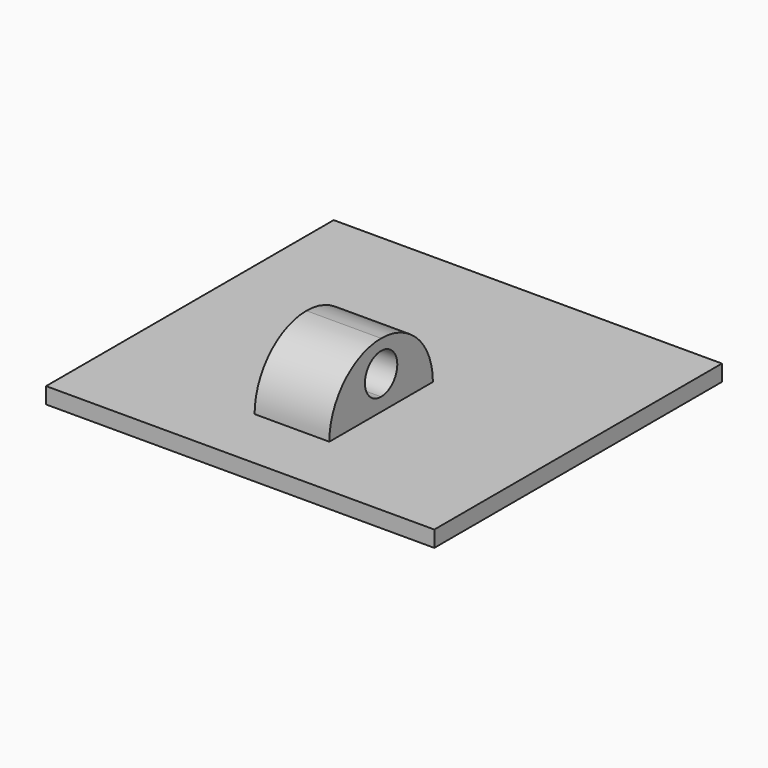
from build123d import *

# Parameters (mm, degrees)
F0_W     = 152.4
F0_H     = 141.1111171471
F1_DEPTH = 6.35
F2_W     = 14.6685
F2_H     = 50.8
F3_DEPTH = 25.4
F4_R     = 25.39999
F6_DEPTH = 76.2


# Not quite as in the source:
# - a fillet or chamfer is up to 0.001 mm smaller than in the source, because OpenCascade refuses the exact size


with BuildPart() as f1:
    # F0 (on Top) → F1 (new body)
    with BuildSketch(Plane.XY):
        Rectangle(F0_W, F0_H)
    extrude(amount=F1_DEPTH)

    # F2 (on face) → F3 (join)
    with BuildSketch(Plane.XY.offset(6.35)):
        with Locations((-7.33425, -19.7555585735)):
            Rectangle(F2_W, F2_H)
        with Locations((7.33425, -19.7555585735)):
            Rectangle(F2_W, F2_H)
    extrude(amount=F3_DEPTH)

    # F4 (radius 25.4 in the source; OpenCascade refuses exactly that, so slightly less here)
    f4_edges = [f1.edges().sort_by_distance(p)[0] for p in [
        (0, 5.644441, 31.75),
        (0, -45.155559, 31.75),
    ]]
    fillet(f4_edges, radius=F4_R)

    # F5 (on face) → F6 (cut)
    with BuildSketch(Plane(origin=(-14.6685, 0, 0), x_dir=(0, -1, 0), z_dir=(-1, 0, 0))):
        with BuildLine():
            Line((19.7555585735, 11.557), (19.7555585735, 27.432))
            ThreePointArc((19.7555585735, 27.432), (11.8180585735, 19.4945), (19.7555585735, 11.557))
        make_face()
        with BuildLine():
            ThreePointArc((27.6930585735, 19.4945), (25.3682186492, 25.1071600757), (19.7555585735, 27.432))
            Line((19.7555585735, 27.432), (19.7555585735, 11.557))
            ThreePointArc((19.7555585735, 11.557), (25.3682186492, 13.8818399243), (27.6930585735, 19.4945))
        make_face()
    extrude(amount=-F6_DEPTH, mode=Mode.SUBTRACT)


solid = f1.part
